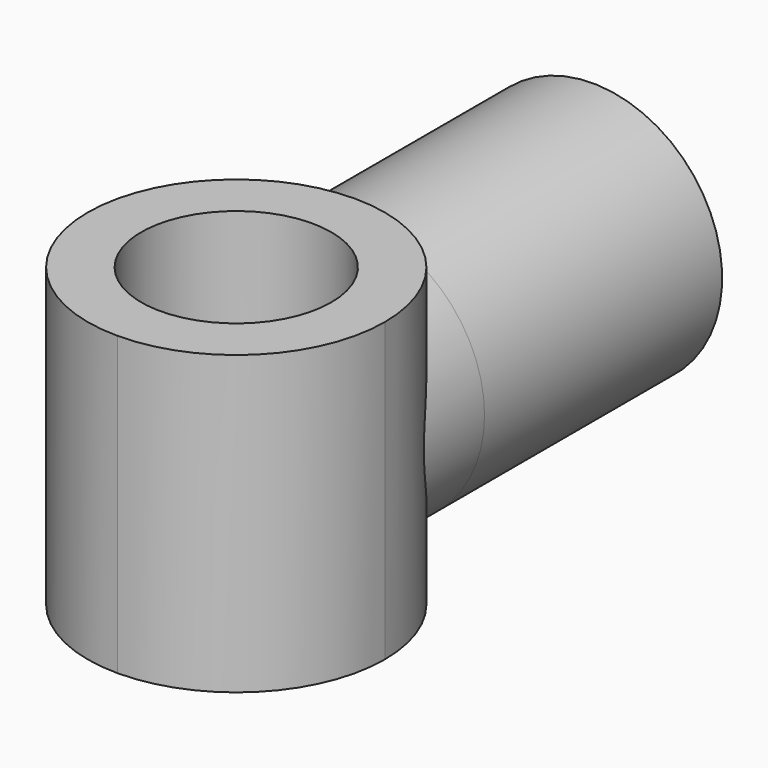
from build123d import *

# Parameters (mm, degrees)
F0_W         = 7.9375
F0_H         = 7.9375
F0_R         = 2.54
F1_DEPTH     = 7.9375
F2_R         = 3.46075
F2_R_2       = 2.54
F3_DEPTH     = 7.9375
F4_T3_DEPTH  = 27.78125
F4_S4_R      = 3.46075
F4_T5_DEPTH  = 16
F4_T8_DEPTH  = 27.78125
F4_S9_R      = 3.46075
F4_T10_DEPTH = 16
F4_T13_DEPTH = 27.78125
F4_T16_DEPTH = 27.78125


# Not quite as in the source:
# - a fillet or chamfer that OpenCascade refuses, or shapes differently, is made with other operations: its cross-section is extruded or revolved along the edge and cut away or added


with BuildPart() as f1:
    # F0 (on Top) → F1 (new body)
    with BuildSketch(Plane.XY):
        Rectangle(F0_W, F0_H)
        Circle(F0_R, mode=Mode.SUBTRACT)
    extrude(amount=F1_DEPTH)

    # F2 (on face) → F3 (join)
    with BuildSketch(Plane(origin=(0, 3.96875, 0), x_dir=(-1, 0, 0), z_dir=(0, 1, 0))):
        with Locations((0, 3.96875)):
            Circle(F2_R)
        with Locations((0, 3.96875)):
            Circle(F2_R_2, mode=Mode.SUBTRACT)
    extrude(amount=F3_DEPTH)

    # F4: fillet of radius 3.96875 on 4 edges, made by hand


with BuildPart() as f4_tool1:
    # F4_s2 → F4_t3 (new body)
    with BuildSketch(Plane.XY.offset(-9.921875)):
        with BuildLine():
            ThreePointArc((0, 3.96875), (-2.8063300378, 2.8063300378), (-3.96875, 0))
            Line((-3.96875, 0), (-3.96875, 3.96875))
            Line((-3.96875, 3.96875), (0, 3.96875))
        make_face()
    extrude(amount=F4_T3_DEPTH)

    # F4_s4 → F4_t5 (cut, symmetric)
    with BuildSketch(Plane.XZ.offset(-2)):
        with Locations((0, 3.96875)):
            Circle(F4_S4_R)
    extrude(amount=F4_T5_DEPTH, both=True, mode=Mode.SUBTRACT)


with BuildPart() as f4_tool6:
    # F4_s7 → F4_t8 (new body)
    with BuildSketch(Plane.XY.offset(-9.921875)):
        with BuildLine():
            ThreePointArc((3.96875, 0), (2.8063300378, 2.8063300378), (0, 3.96875))
            Line((0, 3.96875), (3.96875, 3.96875))
            Line((3.96875, 3.96875), (3.96875, 0))
        make_face()
    extrude(amount=F4_T8_DEPTH)

    # F4_s9 → F4_t10 (cut, symmetric)
    with BuildSketch(Plane.XZ.offset(-2)):
        with Locations((0, 3.96875)):
            Circle(F4_S9_R)
    extrude(amount=F4_T10_DEPTH, both=True, mode=Mode.SUBTRACT)


with BuildPart() as f4_tool11:
    # F4_s12 → F4_t13 (new body)
    with BuildSketch(Plane.XY.offset(-9.921875)):
        with BuildLine():
            ThreePointArc((3.96875, 0), (2.8063300378, -2.8063300378), (0, -3.96875))
            Line((0, -3.96875), (3.96875, -3.96875))
            Line((3.96875, -3.96875), (3.96875, 0))
        make_face()
    extrude(amount=F4_T13_DEPTH)


with BuildPart() as f4_tool14:
    # F4_s15 → F4_t16 (new body)
    with BuildSketch(Plane.XY.offset(-9.921875)):
        with BuildLine():
            ThreePointArc((0, -3.96875), (-2.8063300378, -2.8063300378), (-3.96875, 0))
            Line((-3.96875, 0), (-3.96875, -3.96875))
            Line((-3.96875, -3.96875), (0, -3.96875))
        make_face()
    extrude(amount=F4_T16_DEPTH)


with BuildPart() as f1_1:
    add(f1.part)

    # F4_t17: cut F4_tool1, F4_tool6, F4_tool11, F4_tool14
    add([f4_tool1.part, f4_tool6.part, f4_tool11.part, f4_tool14.part], mode=Mode.SUBTRACT)


solid = f1_1.part
